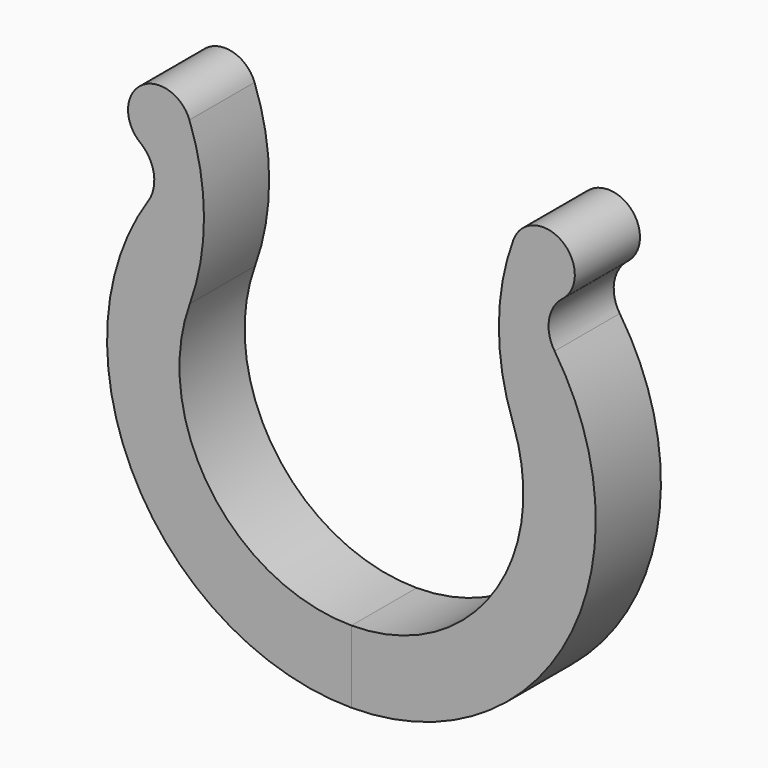
from build123d import *
from build123d import SkipClean  # not in build123d's __all__

# Parameters (mm, degrees)
F1_DEPTH = 0.9


with BuildPart() as f1:
    # F0 (on Front) → F1 (new body)
    with BuildSketch(Plane.XZ):
        with BuildLine():
            ThreePointArc((-1.7854159795, 0.6498382723), (-1.6291374554, 1.5431391957), (-1.7902040585, 2.4355892314))
            ThreePointArc((-1.7902040585, 2.4355892314), (-2.3254361147, 2.5963553546), (-2.3329475668, 2.0375506674))
            ThreePointArc((-2.3329475668, 2.0375506674), (-2.1832734878, 1.7856710143), (-2.2454313543, 1.4993458684))
            ThreePointArc((-2.2454313543, 1.4993458684), (-2.3809907439, -1.2731390645), (0, -2.7))
            Line((0, -2.7), (0, -1.9))
            ThreePointArc((0, -1.9), (-1.5563888841, -1.0897952291), (-1.7854159795, 0.6498382723))
        make_face()
    extrude(amount=F1_DEPTH)

    # F2: F1 across plane


with BuildPart() as f1_1:
    add(f1.part, clean=False)
    with SkipClean():  # cleaning this boolean's faces spoils the solid; the shape is the same uncleaned
        add(f1.part.mirror(Plane.YZ), clean=False)


solid = f1_1.part
